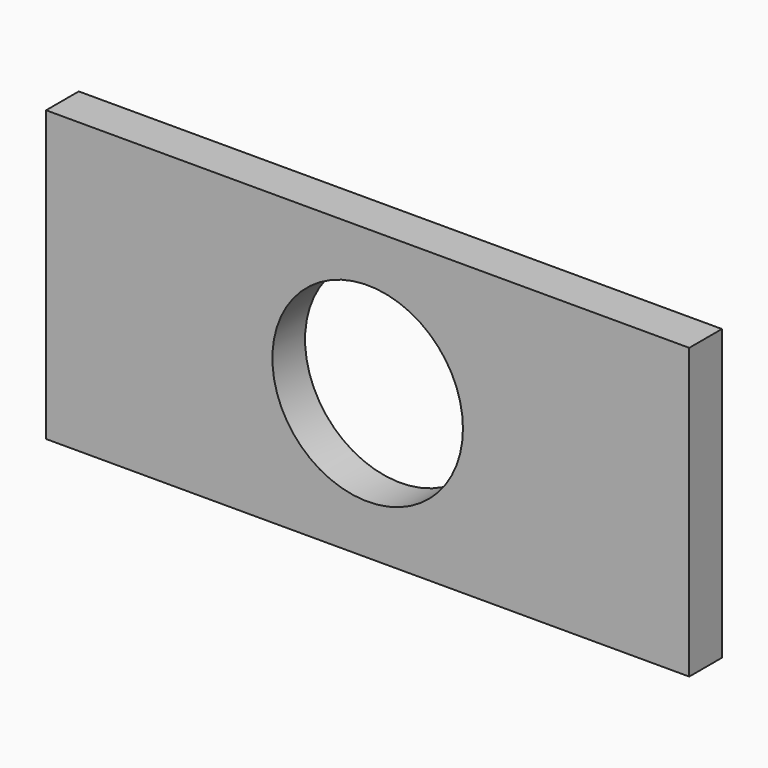
from build123d import *

# Parameters (mm, degrees)
F0_W     = 200
F0_H     = 90
F0_R     = 29.6278920172
F1_DEPTH = 38.1
F2_DEPTH = 25.4


# Not quite as in the source:
# - a feature names something its author has since deleted; it is built from what else it names


with BuildPart() as f1:
    # F0 (on Front) → F1 (new body)
    with BuildSketch(Plane.XZ):
        Rectangle(F0_W, F0_H)
        Circle(F0_R, mode=Mode.SUBTRACT)
    extrude(amount=F1_DEPTH)

    # F2 (cut): a face of the model
    f2_faces = [f1.faces().sort_by_distance(p)[0] for p in [
        (0, -38.1, -42.8068287801),
    ]]
    extrude(f2_faces, amount=-F2_DEPTH, mode=Mode.SUBTRACT)


solid = f1.part
